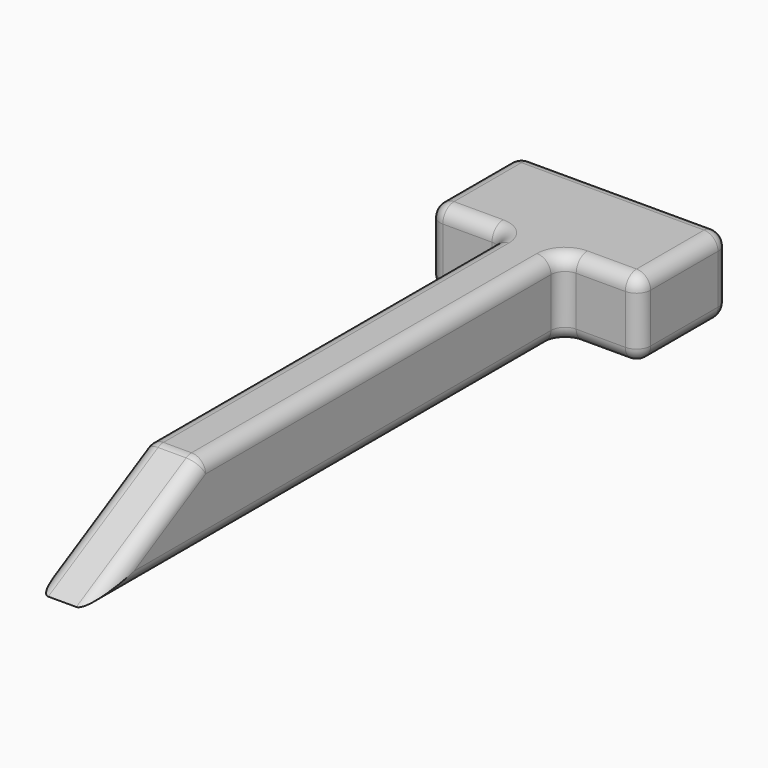
from build123d import *

# Parameters (mm, degrees)
F1_DEPTH = 2
F0_W     = 8
F0_H     = 5.5
F2_DEPTH = 7.5
F4_DEPTH = 5
F5_DEPTH = 0.5
F6_F1_R  = 1
F6_F2_R  = 1


with BuildPart() as f1:
    # F0 (on Right) → F1 (new body, symmetric)
    with BuildSketch(Plane.YZ):
        Polygon((42, 5.5), (10, 5.5), (0, 0), (42, 0), align=None)
    extrude(amount=F1_DEPTH, both=True)

    # F0 (on Right) → F2 (join, symmetric)
    with BuildSketch(Plane.YZ):
        with Locations((46, 2.75)):
            Rectangle(F0_W, F0_H)
    extrude(amount=F2_DEPTH, both=True)

    # F3 (on face) → F4 (cut)
    with BuildSketch(Plane.XY.offset(5.5)):
        with BuildLine():
            ThreePointArc((-2.75, 48.75), (-5.5, 46), (-2.75, 43.25))
            Line((-2.75, 43.25), (2.75, 43.25))
            ThreePointArc((2.75, 43.25), (5.5, 46), (2.75, 48.75))
            Line((2.75, 48.75), (-2.75, 48.75))
        make_face()
    extrude(amount=-F4_DEPTH, mode=Mode.SUBTRACT)

    # F3 (on face) → F5 (join)
    with BuildSketch(Plane.XY.offset(5.5)):
        with BuildLine():
            ThreePointArc((-2.75, 48.75), (-5.5, 46), (-2.75, 43.25))
            Line((-2.75, 43.25), (2.75, 43.25))
            ThreePointArc((2.75, 43.25), (5.5, 46), (2.75, 48.75))
            Line((2.75, 48.75), (-2.75, 48.75))
        make_face()
    extrude(amount=-F5_DEPTH)

    # F6: fillet of radius 1 on 21 edges, made by hand

    # F6_f1
    f6_f1_edges = [f1.edges().sort_by_distance(p)[0] for p in [
        (2, 42, 2.75),
        (-2, 42, 2.75),
    ]]
    fillet(f6_f1_edges, radius=F6_F1_R)

    # F6_f2
    f6_f2_edges = [f1.edges().sort_by_distance(p)[0] for p in [
        (-7.5, 42, 2.75),
        (-7.5, 50, 2.75),
        (7.5, 50, 2.75),
        (7.5, 42, 2.75),
        (-7.5, 46, 5.5),
        (-5.25, 42, 5.5),
        (-2, 25.5, 5.5),
        (0, 10, 5.5),
        (2, 25.5, 5.5),
        (5.25, 42, 5.5),
        (7.5, 46, 5.5),
        (0, 50, 5.5),
        (2, 5, 2.75),
        (2, 20.5, 0),
        (-2, 5, 2.75),
        (-2, 20.5, 0),
        (0, 50, 0),
        (7.5, 46, 0),
        (-7.5, 46, 0),
        (-2.2928932188, 41.7071067812, 0),
        (2.2928932188, 41.7071067812, 0),
        (2.2928932188, 41.7071067812, 5.5),
        (-2.2928932188, 41.7071067812, 5.5),
    ]]
    fillet(f6_f2_edges, radius=F6_F2_R)


solid = f1.part
